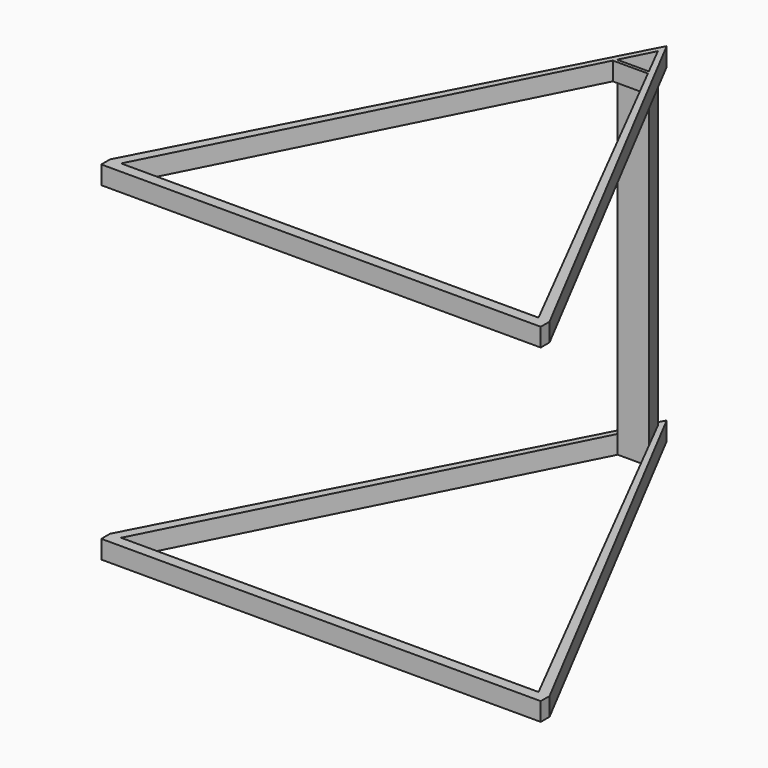
from build123d import *

# Parameters (mm, degrees)
F1_DEPTH      = 5
F3_DEPTH      = 85
F3_DEPTH_BACK = 5
F5_DEPTH      = 5
F7_DEPTH      = 5


# Not quite as in the source:
# - a feature names something its author has since deleted; it is built from what else it names


with BuildPart() as f1:
    # F0 (on Top) → F1 (new body)
    with BuildSketch(Plane.XY):
        Polygon((0, 118), (-60, 3), (-57, 3), (0, 115), (57, 3), (60, 3), align=None)
        Polygon((-60, 0), (0, 0), (60, 0), (60, 3), (57, 3), (-57, 3), (-60, 3), align=None)
    extrude(amount=F1_DEPTH)

    # F2 (on face) → F3 (join, two sides)
    with BuildSketch(Plane.XY.offset(5)) as f3_sk:
        Polygon((-4.2687140089, 106.6123514211), (4.2687140089, 106.6123514211), (0, 115), align=None)
    extrude(amount=F3_DEPTH)
    extrude(f3_sk.sketch, amount=-F3_DEPTH_BACK)


with BuildPart() as f5:
    # F4 (on face) → F5 (new body)
    with BuildSketch(Plane.XY.offset(90)):
        Polygon((0, 118), (0, 115), (4.2687140089, 106.6123514211), (56.999907785, 3.0001811943), (59.999907785, 3.0001811943), align=None)
        Polygon((-4.2687140089, 106.6123514211), (0, 115), (0, 118), (-59.999907785, 3.0001811943), (-56.999907785, 3.0001811943), align=None)
        Polygon((56.999907785, 3.0001811943), (-56.999907785, 3.0001811943), (-59.999907785, 3.0001811943), (-59.999907785, 0.0001811943), (59.999907785, 0.0001811943), (59.999907785, 3.0001811943), align=None)
    extrude(amount=F5_DEPTH)

    # F6 (on face) → F7 (join)
    with BuildSketch(Plane(origin=(0, 0, 90), x_dir=(1, 0, 0), z_dir=(0, 0, -1))):
        Polygon((-4.782894762, -105.6020313448), (-4.3293266249, -106.4932529475), (4.3293266249, -106.4932529475), (4.782894762, -105.6020313448), align=None)
    extrude(amount=-F7_DEPTH)


solid = Compound([f1.part, f5.part])
